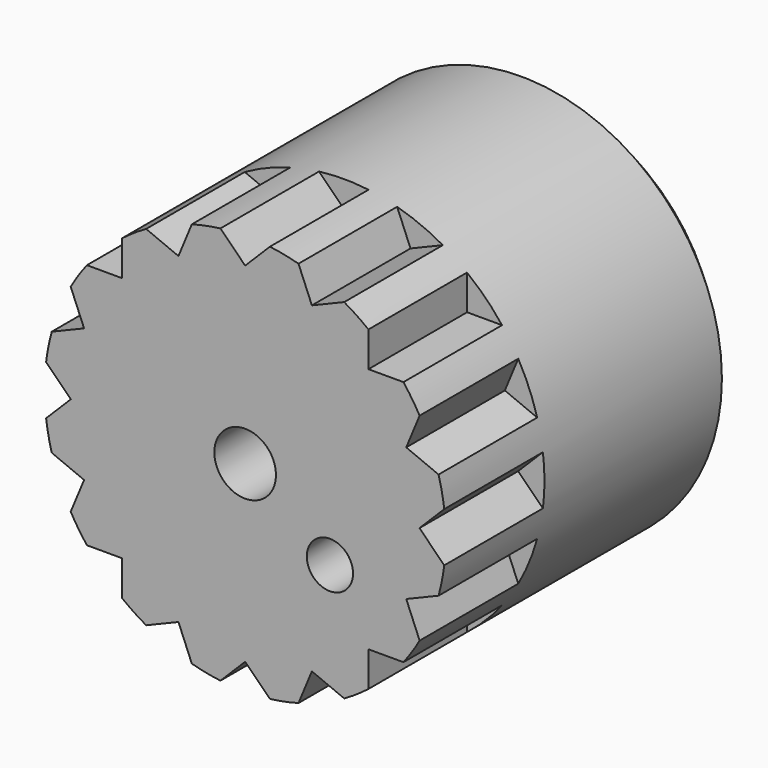
from build123d import *

# Parameters (mm, degrees)
F0_R            = 41.3322868319
F1_DEPTH        = 76.2
F2_W            = 25.4
F2_H            = 25.4
F3_DEPTH        = 25.4
F3_COPIES_COUNT = 16
F4_SIZE         = 5.08
F6_D            = 12.7
F7_R            = 4.7625
F8_DEPTH        = 76.2


# Not quite as in the source:
# - a pattern or mirror of a feature is missing from the dataset's text; its kind, count and spacing are read off the source's solid


with BuildPart() as f1:
    # F0 (on Front) → F1 (new body)
    with BuildSketch(Plane.XZ):
        Circle(F0_R)
    extrude(amount=F1_DEPTH)

    # F2 (on face) → F3 (cut)
    with BuildSketch(Plane.XZ.offset(76.2)):
        with Locations((38.1, 38.1)):
            Rectangle(F2_W, F2_H)
    f3 = extrude(amount=-F3_DEPTH, mode=Mode.SUBTRACT)

    # F3_copies: F3 ×16 about axis
    f3_copies_axis = Axis((0, 0, 0), (0, 1, 0))
    for i in range(1, F3_COPIES_COUNT):
        add(f3.rotate(f3_copies_axis, i * 360 / F3_COPIES_COUNT), mode=Mode.SUBTRACT)

    # F4
    f4_edges = [f1.edges().sort_by_distance(p)[0] for p in [
        (-41.332287, 0, 0),
    ]]
    chamfer(f4_edges, length=F4_SIZE)

    # F6 (through all)
    with Locations(Plane.XZ.offset(76.2)):
        with Locations((0, 0)):
            Hole(F6_D / 2)

    # F7 (on face) → F8 (cut, through all)
    with BuildSketch(Plane.XZ.offset(76.2)):
        with Locations((17.4625, -12.6960306297)):
            Circle(F7_R)
    extrude(amount=-F8_DEPTH, mode=Mode.SUBTRACT)


solid = f1.part
